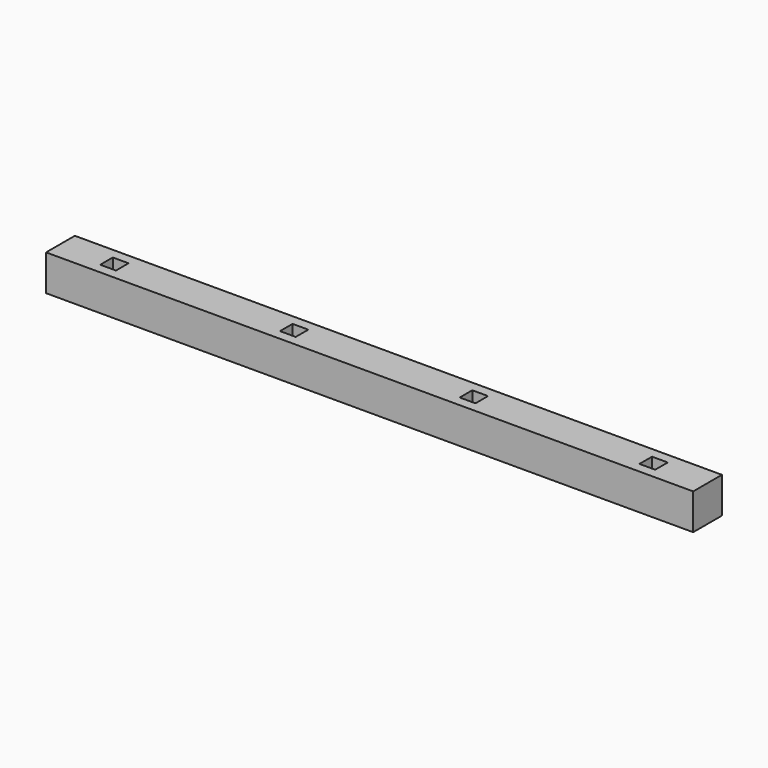
from build123d import *

# Parameters (mm, degrees)
F0_W            = 101.6
F0_H            = 101.6
F1_DEPTH        = 914.4
F2_W            = 44.45
F2_H            = 44.45
F3_DEPTH        = 101.601
F4_W            = 44.45
F4_H            = 44.45
F5_DEPTH        = 101.601
F5_COPIES_COUNT = 3
F5_COPIES_PITCH = 508


# Not quite as in the source:
# - a pattern or mirror of a feature is missing from the dataset's text; its kind, count and spacing are read off the source's solid


with BuildPart() as f1:
    # F0 (on Right) → F1 (new body, symmetric)
    with BuildSketch(Plane.YZ):
        Rectangle(F0_W, F0_H)
    extrude(amount=F1_DEPTH, both=True)

    # F2 (on face) → F3 (cut, through all)
    with BuildSketch(Plane.XY.offset(50.8)):
        with Locations((-762, 0)):
            Rectangle(F2_W, F2_H)
    extrude(amount=-F3_DEPTH, mode=Mode.SUBTRACT)

    # F4 (on face) → F5 (cut, through all)
    with BuildSketch(Plane.XY.offset(50.8)):
        with Locations((-254, 0)):
            Rectangle(F4_W, F4_H)
    f5 = extrude(amount=-F5_DEPTH, mode=Mode.SUBTRACT)

    # F5_copies: F5 ×3
    with Locations(*[(i * F5_COPIES_PITCH, 0, 0) for i in range(1, F5_COPIES_COUNT)]):
        add(f5, mode=Mode.SUBTRACT)


solid = f1.part
